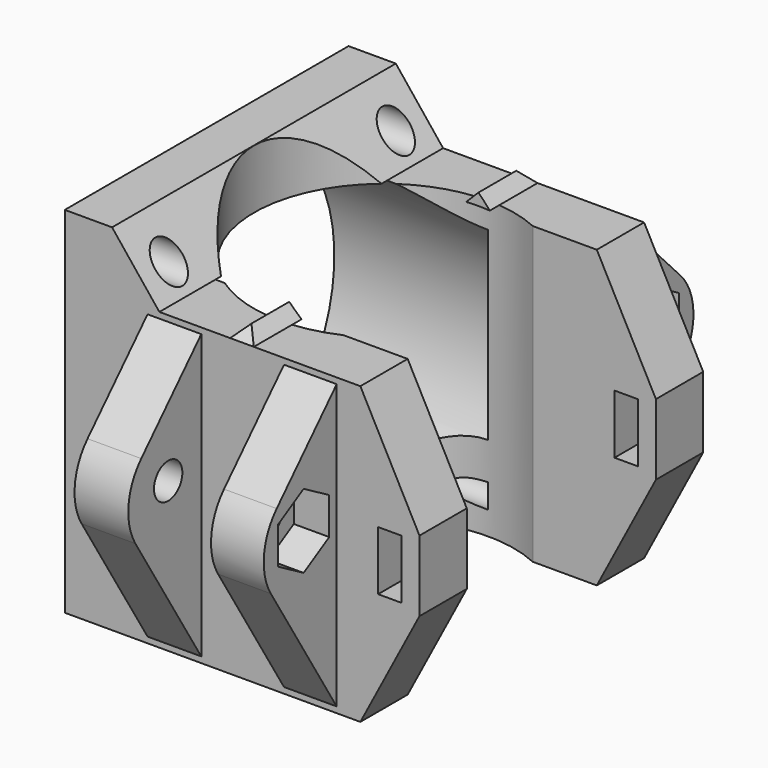
from build123d import *

# Parameters (mm, degrees)
F0_W      = 2
F0_H      = 5
F5_DEPTH  = 15
F6_DEPTH  = 15
F7_DEPTH  = 16
F2_R      = 1.43
F8_DEPTH  = 25
F9_DEPTH  = 25
F3_R      = 1.5
F10_DEPTH = 8
F11_START = 5
F11_DEPTH = 20
F4_W      = 7
F4_H      = 12
F12_DEPTH = 20
F14_START = 10
F13_W     = 2
F13_H     = 30
F14_DEPTH = 1
F15_R     = 10
F16_DEPTH = 25
F17_SIZE  = 0.9999


# Not quite as in the source:
# - a fillet or chamfer is up to 0.001 mm smaller than in the source, because OpenCascade refuses the exact size


with BuildPart() as f5:
    # F0 (on Front) → F5 (new body, symmetric)
    with BuildSketch(Plane.XZ):
        Polygon((-11, 15), (-15, 15), (-15, -15), (10, -15), (10, 10), (-7, 10), align=None)
        Polygon((10, 10), (10, -15), (15, -5.5), (15, 0.5), align=None)
        with Locations((12.5, -2.5)):
            Rectangle(F0_W, F0_H, mode=Mode.SUBTRACT)
    extrude(amount=F5_DEPTH, both=True)

    # F1 (on Top) → F6 (cut, symmetric)
    with BuildSketch(Plane.XY):
        with BuildLine():
            Line((16, 10), (4.582575695, 10))
            ThreePointArc((4.582575695, 10), (-11, 0), (4.582575695, -10))
            Line((4.582575695, -10), (16, -10))
            Line((16, -10), (16, 10))
        make_face()
    extrude(amount=F6_DEPTH, both=True, mode=Mode.SUBTRACT)

    # F2 (on Right) → F7 (cut)
    with BuildSketch(Plane.YZ):
        with BuildLine():
            Line((9.0691785736, 10), (-9.0691785736, 10))
            ThreePointArc((-9.0691785736, 10), (0, -13.5), (9.0691785736, 10))
        make_face()
    extrude(amount=-F7_DEPTH, mode=Mode.SUBTRACT)

    # F2 (on Right) → F8 (cut)
    with BuildSketch(Plane.YZ):
        with Locations((12, 12)):
            Circle(F2_R)
        with Locations((-12, 12)):
            Circle(F2_R)
    extrude(amount=-F8_DEPTH, mode=Mode.SUBTRACT)

    # F2 (on Right) → F9 (cut)
    with BuildSketch(Plane.YZ):
        with Locations((12, -12)):
            Circle(F2_R)
        with Locations((-12, -12)):
            Circle(F2_R)
    extrude(amount=-F9_DEPTH, mode=Mode.SUBTRACT)

    # F3 (on Right) → F10 (join, symmetric)
    with BuildSketch(Plane.YZ):
        with BuildLine():
            Line((15, -14.5), (21.9673867507, -3.2620052331))
            ThreePointArc((21.9673867507, -3.2620052331), (22.6917908233, -0.1175906407), (21.3446249631, 2.8145158605))
            Line((21.3446249631, 2.8145158605), (15, 9.5))
            Line((15, 9.5), (15, -14.5))
        make_face()
        Polygon((18.5, 3.129238459), (21.21, 1.5646192295), (21.21, -1.5646192295), (18.5, -3.129238459), (15.79, -1.5646192295), (15.79, 1.5646192295), align=None, mode=Mode.SUBTRACT)
        Polygon((21.21, -1.5646192295), (21.21, 1.5646192295), (18.5, 3.129238459), (15.79, 1.5646192295), (15.79, -1.5646192295), (18.5, -3.129238459), align=None)
        with Locations((18.5, 0)):
            Circle(F3_R, mode=Mode.SUBTRACT)
        with BuildLine():
            Line((-15, 9.5), (-21.3446249631, 2.8145158605))
            ThreePointArc((-21.3446249631, 2.8145158605), (-22.6917908233, -0.1175906407), (-21.9673867507, -3.2620052331))
            Line((-21.9673867507, -3.2620052331), (-15, -14.5))
            Line((-15, -14.5), (-15, 9.5))
        make_face()
        Polygon((-21.21, 1.5646192295), (-18.5, 3.129238459), (-15.79, 1.5646192295), (-15.79, -1.5646192295), (-18.5, -3.129238459), (-21.21, -1.5646192295), align=None, mode=Mode.SUBTRACT)
        Polygon((-15.79, 1.5646192295), (-18.5, 3.129238459), (-21.21, 1.5646192295), (-21.21, -1.5646192295), (-18.5, -3.129238459), (-15.79, -1.5646192295), align=None)
        with Locations((-18.5, 0)):
            Circle(F3_R, mode=Mode.SUBTRACT)
    extrude(amount=F10_DEPTH, both=True)

    # F3 (on Right) → F11 (cut)
    with BuildSketch(Plane.YZ.offset(F11_START)):
        Polygon((21.21, -1.5646192295), (21.21, 1.5646192295), (18.5, 3.129238459), (15.79, 1.5646192295), (15.79, -1.5646192295), (18.5, -3.129238459), align=None)
        with Locations((18.5, 0)):
            Circle(F3_R, mode=Mode.SUBTRACT)
        with Locations((18.5, 0)):
            Circle(F3_R)
        Polygon((-15.79, 1.5646192295), (-18.5, 3.129238459), (-21.21, 1.5646192295), (-21.21, -1.5646192295), (-18.5, -3.129238459), (-15.79, -1.5646192295), align=None)
        with Locations((-18.5, 0)):
            Circle(F3_R, mode=Mode.SUBTRACT)
        with Locations((-18.5, 0)):
            Circle(F3_R)
    extrude(amount=F11_DEPTH, mode=Mode.SUBTRACT)

    # F4 (on Top) → F12 (cut, symmetric)
    with BuildSketch(Plane.XY):
        with Locations((0.0437486451, 21)):
            Rectangle(F4_W, F4_H)
        with Locations((0.0437486451, -21)):
            Rectangle(F4_W, F4_H)
    extrude(amount=F12_DEPTH, both=True, mode=Mode.SUBTRACT)

    # F13 (on Top) → F14 (join)
    with BuildSketch(Plane.XY.offset(F14_START)):
        with Locations((-0.0117724412, 0)):
            Rectangle(F13_W, F13_H)
    extrude(amount=F14_DEPTH)

    # F15 (on Top) → F16 (cut)
    with BuildSketch(Plane.XY):
        Circle(F15_R)
    extrude(amount=F16_DEPTH, mode=Mode.SUBTRACT)

    # F17 (size 1 in the source; OpenCascade refuses exactly that, so slightly less here)
    f17_edges = [f5.edges().sort_by_distance(p)[0] for p in [
        (0.988228, 12.475525, 11),
        (-1.011772, 12.474342, 11),
        (-0.011772, 15, 11),
        (0.988228, -12.475525, 11),
        (-0.011772, -15, 11),
        (-1.011772, -12.474342, 11),
    ]]
    chamfer(f17_edges, length=F17_SIZE)


solid = f5.part
